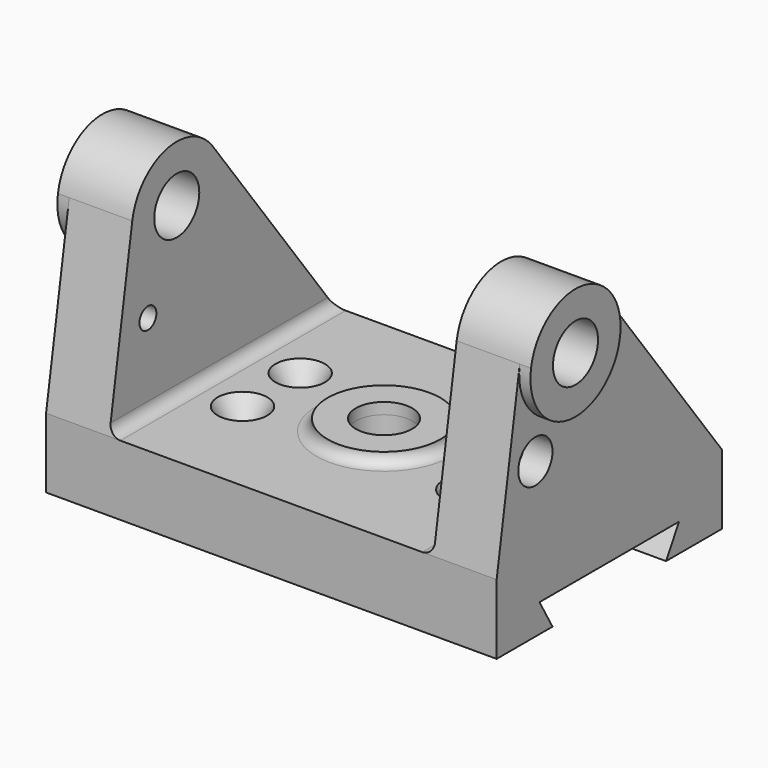
from build123d import *

# Parameters (mm, degrees)
F0_R            = 6.35
F1_DEPTH        = 50.8
F2_DEPTH        = 53.34
F3_DEPTH        = 36.576
F5_D            = 4.7752
F5_CSINK_D      = 11.176
F5_CSINK_ANGLE  = 60
F4_R            = 6.35
F6_DEPTH        = 25.4
F4_R_2          = 12.7
F7_DEPTH        = 2.54
F8_R            = 2.53999
F10_D           = 4.7752
F10_DEPTH       = 25.4
F10_CBORE_D     = 9.652
F10_CBORE_DEPTH = 6.35
F10_TIP         = 1.434614814
F12_D           = 4.7752
F12_DEPTH       = 25.4
F12_CBORE_D     = 9.652
F12_CBORE_DEPTH = 6.35
F12_TIP         = 1.434614814


# Not quite as in the source:
# - a fillet or chamfer is up to 0.001 mm smaller than in the source, because OpenCascade refuses the exact size


with BuildPart() as f1:
    # F0 (on Right) → F1 (new body, symmetric)
    with BuildSketch(Plane.YZ):
        with BuildLine():
            ThreePointArc((-25.2359570421, 40.1346451877), (-13.7206237225, 25.44107717), (0, 38.1))
            ThreePointArc((0, 38.1), (-0.6517221148, 42.1160926284), (-2.54, 45.72))
            ThreePointArc((-2.54, 45.72), (-15.7348542076, 50.4320582199), (-25.2359570421, 40.1346451877))
        make_face()
        with Locations((-12.7, 38.1)):
            Circle(F0_R, mode=Mode.SUBTRACT)
        with BuildLine():
            ThreePointArc((-2.54, 45.72), (-0.6517221148, 42.1160926284), (0, 38.1))
            ThreePointArc((0, 38.1), (-13.7206237225, 25.44107717), (-25.2359570421, 40.1346451877))
            Line((-25.2359570421, 40.1346451877), (-31.75, 0))
            Line((-31.75, 0), (31.75, 0))
            Line((31.75, 0), (-2.54, 45.72))
        make_face()
        Polygon((31.75, -15.748), (31.75, 0), (-31.75, 0), (-31.75, -15.748), (-16.002, -15.748), (-19.6681742094, -9.398), (19.6681742094, -9.398), (16.002, -15.748), align=None)
    extrude(amount=F1_DEPTH, both=True)

    # F0 (on Right) → F2 (join, symmetric)
    with BuildSketch(Plane.YZ):
        with BuildLine():
            ThreePointArc((-25.2359570421, 40.1346451877), (-13.7206237225, 25.44107717), (0, 38.1))
            ThreePointArc((0, 38.1), (-0.6517221148, 42.1160926284), (-2.54, 45.72))
            ThreePointArc((-2.54, 45.72), (-15.7348542076, 50.4320582199), (-25.2359570421, 40.1346451877))
        make_face()
        with Locations((-12.7, 38.1)):
            Circle(F0_R, mode=Mode.SUBTRACT)
    extrude(amount=F2_DEPTH, both=True)

    # F0 (on Right) → F3 (cut, symmetric)
    with BuildSketch(Plane.YZ):
        with BuildLine():
            ThreePointArc((-2.54, 45.72), (-0.6517221148, 42.1160926284), (0, 38.1))
            ThreePointArc((0, 38.1), (-13.7206237225, 25.44107717), (-25.2359570421, 40.1346451877))
            Line((-25.2359570421, 40.1346451877), (-31.75, 0))
            Line((-31.75, 0), (31.75, 0))
            Line((31.75, 0), (-2.54, 45.72))
        make_face()
        with BuildLine():
            ThreePointArc((-25.2359570421, 40.1346451877), (-13.7206237225, 25.44107717), (0, 38.1))
            ThreePointArc((0, 38.1), (-0.6517221148, 42.1160926284), (-2.54, 45.72))
            ThreePointArc((-2.54, 45.72), (-15.7348542076, 50.4320582199), (-25.2359570421, 40.1346451877))
        make_face()
        with Locations((-12.7, 38.1)):
            Circle(F0_R, mode=Mode.SUBTRACT)
    extrude(amount=F3_DEPTH, both=True, mode=Mode.SUBTRACT)

    # F5 (through all)
    with Locations(Plane.XY):
        with Locations((-25.4, 8.128), (-25.4, -8.128), (25.4, 8.128), (25.4, -8.128)):
            CounterSinkHole(F5_D / 2, F5_CSINK_D / 2, counter_sink_angle=F5_CSINK_ANGLE)

    # F4 (on face) → F6 (cut)
    with BuildSketch(Plane.XY):
        Circle(F4_R)
    extrude(amount=-F6_DEPTH, mode=Mode.SUBTRACT)

    # F4 (on face) → F7 (join)
    with BuildSketch(Plane.XY):
        Circle(F4_R_2)
        Circle(F4_R, mode=Mode.SUBTRACT)
    extrude(amount=F7_DEPTH)

    # F8 (radius 2.54 in the source; OpenCascade refuses exactly that, so slightly less here)
    f8_edges = [f1.edges().sort_by_distance(p)[0] for p in [
        (-12.7, 0, 0),
        (36.576, 0, 0),
        (-36.576, 0, 0),
    ]]
    fillet(f8_edges, radius=F8_R)

    # F10
    with Locations(Plane.YZ.offset(50.8)):
        with Locations((-20.828, 19.05)):
            CounterBoreHole(F10_D / 2, F10_CBORE_D / 2, F10_CBORE_DEPTH, depth=F10_DEPTH)
            with Locations((0, 0, -(F10_DEPTH + F10_TIP / 2))):  # 118° drill point
                Cone(0, F10_D / 2, F10_TIP, mode=Mode.SUBTRACT)

    # F12
    with Locations(Plane(origin=(-50.8, 0, 0), x_dir=(0, -1, 0), z_dir=(-1, 0, 0))):
        with Locations((20.828, 19.05)):
            CounterBoreHole(F12_D / 2, F12_CBORE_D / 2, F12_CBORE_DEPTH, depth=F12_DEPTH)
            with Locations((0, 0, -(F12_DEPTH + F12_TIP / 2))):  # 118° drill point
                Cone(0, F12_D / 2, F12_TIP, mode=Mode.SUBTRACT)


solid = f1.part
